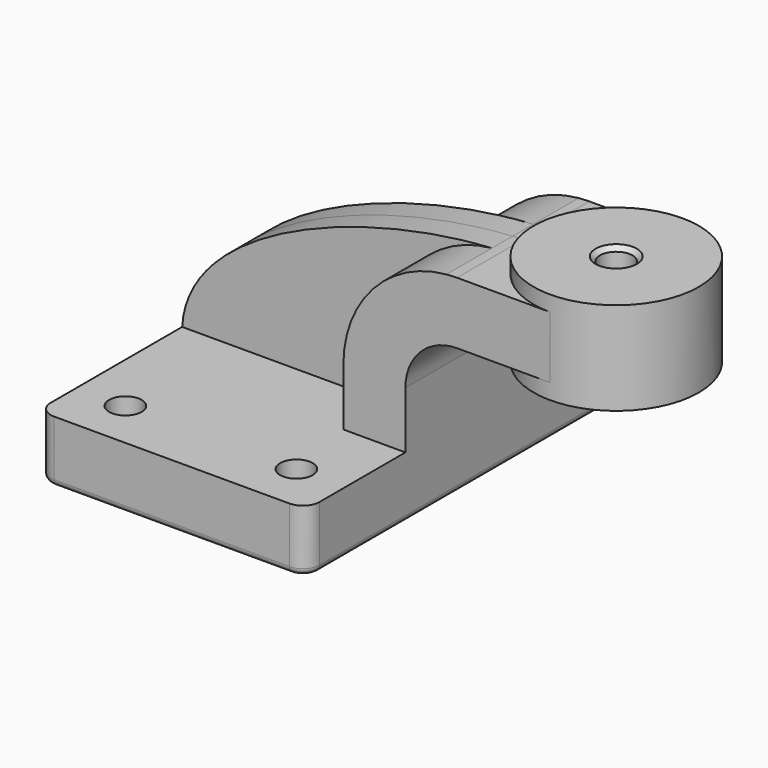
from build123d import *

# Parameters (mm, degrees)
F1_DEPTH        = 63.5
F0_W            = 25.4
F0_H            = 19.05
F2_DEPTH        = 25.4
F3_DEPTH        = 7.9375
F5_R            = 5.08
F6_R            = 2
F7_R            = 5
F8_DEPTH        = 19.051
F10_D           = 10
F10_CSINK_D     = 12.7
F10_CSINK_ANGLE = 90


# Not quite as in the source:
# - a pattern or mirror of a feature is missing from the dataset's text; its kind, count and spacing are read off the source's solid


with BuildPart() as f1:
    # F0 (on Front) → F1 (new body, symmetric)
    with BuildSketch(Plane.XZ):
        Polygon((22.225, 9.525), (-41.275, 9.525), (-41.275, -9.525), (41.275, -9.525), (41.275, 9.525), align=None)
    extrude(amount=F1_DEPTH, both=True)

    # F0 (on Front) → F2 (join, symmetric)
    with BuildSketch(Plane.XZ):
        with BuildLine():
            Line((22.225, 27.0002), (22.225, 9.525))
            Line((22.225, 9.525), (41.275, 9.525))
            Line((41.275, 9.525), (41.275, 27.0002))
            ThreePointArc((41.275, 27.0002), (45.9246798487, 38.2255201513), (57.15, 42.8752))
            Line((57.15, 42.8752), (60.325, 42.8752))
            Line((60.325, 42.8752), (60.325, 61.9252))
            Line((60.325, 61.9252), (57.15, 61.9252))
            add(Edge.make_bspline(
                [(53.8854342407, 61.7722898912), (54.9842067368, 61.8365871986), (56.0728453275, 61.8876096574), (57.15, 61.9252)],
                knots=[108.5245810491, 108.5245810491, 108.5245810491, 108.5245810491, 111.5045361635, 111.5045361635, 111.5045361635, 111.5045361635], degree=3))
            ThreePointArc((53.8854342407, 61.7722898912), (31.3258777096, 50.5133948686), (22.225, 27.0002))
        make_face()
        with Locations((73.025, 52.4002)):
            Rectangle(F0_W, F0_H)
    extrude(amount=F2_DEPTH, both=True)

    # F0 (on Front) → F3 (join, symmetric)
    with BuildSketch(Plane.XZ):
        with BuildLine():
            add(Edge.make_bspline(
                [(-41.275, 9.525), (-39.5856284224, 39.4828766469), (13.870125209, 59.4306981306), (53.8854342407, 61.7722898912)],
                knots=[0, 0, 0, 0, 108.5245810491, 108.5245810491, 108.5245810491, 108.5245810491], degree=3))
            Line((-41.275, 9.525), (22.225, 9.525))
            Line((22.225, 9.525), (22.225, 27.0002))
            ThreePointArc((22.225, 27.0002), (31.3258777096, 50.5133948686), (53.8854342407, 61.7722898912))
        make_face()
    extrude(amount=F3_DEPTH, both=True)

    # F0 (on Front) → F4 (revolve)
    with BuildSketch(Plane.XZ):
        Polygon((85.725, 66.675), (85.725, 61.9252), (85.725, 42.8752), (85.725, 38.1), (111.125, 38.1), (111.125, 66.675), align=None)
    revolve(axis=Axis((85.725, 0, 52.3875), (0, 0, 1)))

    # F5
    f5_edges = [f1.edges().sort_by_distance(p)[0] for p in [
        (41.275, -63.5, 0),
        (-41.275, -63.5, 0),
        (41.275, 63.5, 0),
        (-41.275, 63.5, 0),
    ]]
    fillet(f5_edges, radius=F5_R)

    # F6
    f6_edges = [f1.edges().sort_by_distance(p)[0] for p in [
        (0, 63.5, -9.525),
        (41.275, 0, -9.525),
        (39.787102, 62.012102, -9.525),
        (-39.787102, 62.012102, -9.525),
        (-41.275, 0, -9.525),
        (-39.787102, -62.012102, -9.525),
        (0, -63.5, -9.525),
        (39.787102, -62.012102, -9.525),
    ]]
    fillet(f6_edges, radius=F6_R)

    # F7 (on face) → F8 (cut, through all)
    with BuildSketch(Plane.XY.offset(9.525)):
        with Locations((-26.275, 48.5)):
            Circle(F7_R)
        with Locations((26.275, 48.5)):
            Circle(F7_R)
    f8 = extrude(amount=-F8_DEPTH, mode=Mode.SUBTRACT)

    # F8_copies: F8 across plane
    add(f8.mirror(Plane(origin=(0, 0, 0), x_dir=(0, 0, -1), z_dir=(0, -1, 0))), mode=Mode.SUBTRACT)

    # F10 (through all)
    with Locations(Plane.XY.offset(66.675)):
        with Locations((85.725, 0)):
            CounterSinkHole(F10_D / 2, F10_CSINK_D / 2, counter_sink_angle=F10_CSINK_ANGLE)


solid = f1.part
